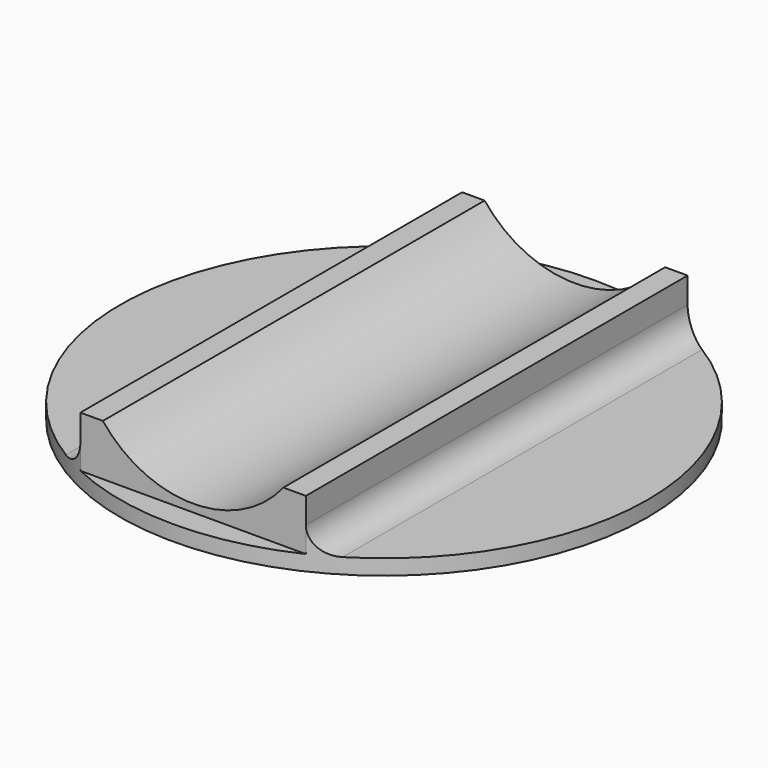
from build123d import *

# Parameters (mm, degrees)
F0_R        = 51.5
F1_DEPTH    = 3
F2_W        = 44
F2_H        = 93.1289428696
F3_DEPTH    = 10
F5_DEPTH    = 93.1289428696
F6_T4_DEPTH = 93.1289428696
F6_S5_R     = 51.5
F6_T6_DEPTH = 48
F7_T4_DEPTH = 93.1289428696
F7_S5_R     = 51.5
F7_T6_DEPTH = 48


# Not quite as in the source:
# - a fillet or chamfer that OpenCascade refuses, or shapes differently, is made with other operations: its cross-section is extruded or revolved along the edge and cut away or added


with BuildPart() as f1:
    # F0 (on Top) → F1 (new body)
    with BuildSketch(Plane.XY):
        Circle(F0_R)
    extrude(amount=F1_DEPTH)

    # F2 (on face) → F3 (join)
    with BuildSketch(Plane.XY.offset(3)):
        Rectangle(F2_W, F2_H)
    extrude(amount=F3_DEPTH)

    # F4 (on face) → F5 (cut, through all)
    with BuildSketch(Plane(origin=(0, 46.5644714348, 0), x_dir=(-1, 0, 0), z_dir=(0, 1, 0))):
        with BuildLine():
            Line((17.6139149538, 13), (-17.6139149538, 13))
            ThreePointArc((-17.6139149538, 13), (0, 4.5), (17.6139149538, 13))
        make_face()
    extrude(amount=-F5_DEPTH, mode=Mode.SUBTRACT)

    # F6: fillet of radius 5 on 1 edges, made by hand


with BuildPart() as f6_tool2:
    # F6_s3 → F6_t4 (new body)
    with BuildSketch(Plane.XZ.offset(-46.5644714348)):
        with BuildLine():
            ThreePointArc((-27, 3), (-23.4644660941, 4.4644660941), (-22, 8))
            Line((-22, 8), (-22, 3))
            Line((-22, 3), (-27, 3))
        make_face()
    extrude(amount=F6_T4_DEPTH)

    # F6_s5 → F6_t6 (intersect, symmetric)
    with BuildSketch(Plane.XY.offset(5.5)):
        Circle(F6_S5_R)
    extrude(amount=F6_T6_DEPTH, both=True, mode=Mode.INTERSECT)


with BuildPart() as f1_1:
    add(f1.part)

    # F6_t1: union F6_tool2
    add(f6_tool2.part)

    # F7: fillet of radius 5 on 1 edges, made by hand


with BuildPart() as f7_tool2:
    # F7_s3 → F7_t4 (new body)
    with BuildSketch(Plane.XZ.offset(46.5644714348)):
        with BuildLine():
            ThreePointArc((27, 3), (23.4644660941, 4.4644660941), (22, 8))
            Line((22, 8), (22, 3))
            Line((22, 3), (27, 3))
        make_face()
    extrude(amount=-F7_T4_DEPTH)

    # F7_s5 → F7_t6 (intersect, symmetric)
    with BuildSketch(Plane.XY.offset(5.5)):
        Circle(F7_S5_R)
    extrude(amount=F7_T6_DEPTH, both=True, mode=Mode.INTERSECT)


with BuildPart() as f1_2:
    add(f1_1.part)

    # F7_t1: union F7_tool2
    add(f7_tool2.part)


solid = f1_2.part
